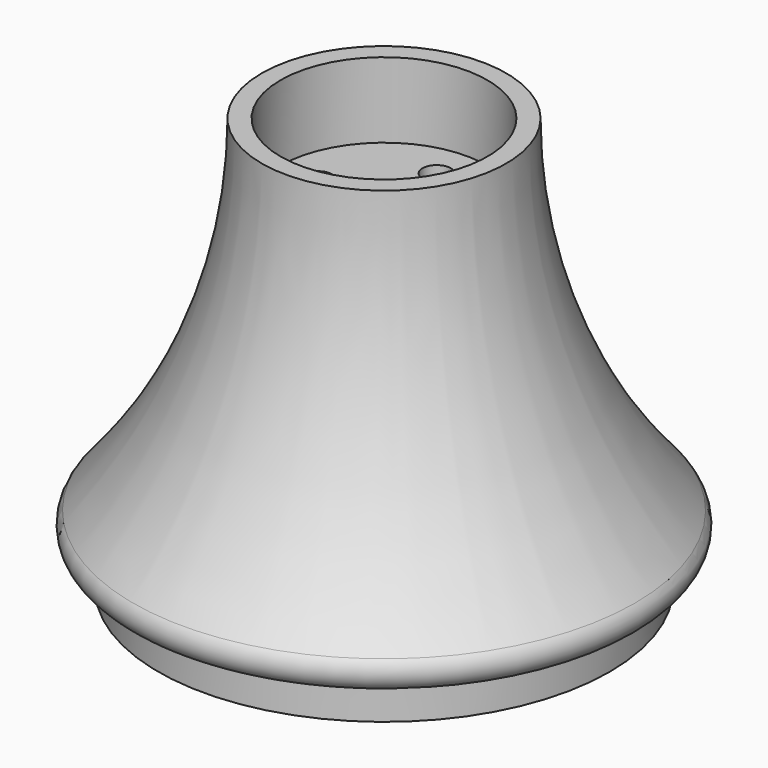
from build123d import *

# Parameters (mm, degrees)
F0_W            = 558.8
F0_H            = 152.4
F2_R            = 152.4
F2_R_2          = 76.2
F3_DEPTH        = 152.4
F3_COPIES_COUNT = 4
F6_DEPTH        = 254


# Not quite as in the source:
# - a pattern or mirror of a feature is missing from the dataset's text; its kind, count and spacing are read off the source's solid


with BuildPart() as f1:
    # F0 (on Front) → F1 (revolve)
    with BuildSketch(Plane.XZ):
        with BuildLine():
            Line((-558.8, -406.4), (-558.8, 0))
            Line((-558.8, 0), (-660.4, 0))
            ThreePointArc((-660.4, 0), (-789.186679788, -846.2615933806), (-1163.8861392232, -1615.9011248632))
            Line((-1163.8861392232, -1615.9011248632), (-1016, -1676.4))
            Line((-1016, -1676.4), (-558.8, -558.8))
            Line((-558.8, -558.8), (-558.8, -406.4))
        make_face()
        with Locations((-279.4, -482.6)):
            Rectangle(F0_W, F0_H)
        with BuildLine():
            Line((-1016, -1676.4), (-1163.8861392232, -1615.9011248632))
            ThreePointArc((-1163.8861392232, -1615.9011248632), (-1256.5295136119, -1742.5177427065), (-1356.0122322887, -1863.8344827586))
            ThreePointArc((-1356.0122322887, -1863.8344827586), (-1371.6828397721, -1972.5871037657), (-1279.255526299, -2032))
            Line((-1279.255526299, -2032), (-1219.2, -2032))
            Line((-1219.2, -2032), (-1219.2, -2235.2))
            Line((-1219.2, -2235.2), (-1016, -2235.2))
            Line((-1016, -2235.2), (-1016, -1676.4))
        make_face()
    revolve(axis=Axis((0, 0, -482.6), (0, 0, -1)))

    # F2 (on face) → F3 (cut)
    with BuildSketch(Plane.XY.offset(-406.4)):
        Circle(F2_R)
        with Locations((0, 355.6)):
            Circle(F2_R_2)
    f3 = extrude(amount=-F3_DEPTH, mode=Mode.SUBTRACT)

    # F3_copies: F3 ×4 about axis
    f3_copies_axis = Axis((0, 0, 0), (0, 0, 1))
    for i in range(1, F3_COPIES_COUNT):
        add(f3.rotate(f3_copies_axis, i * 360 / F3_COPIES_COUNT), mode=Mode.SUBTRACT)

    # F5 (on line) → F6 (cut)
    with BuildSketch(Plane(origin=(-430.7477321435, 0, 176.2149813314), x_dir=(0, -1, 0), z_dir=(-0.9255469562, 0, 0.3786328457))):
        with BuildLine():
            Line((224.0073072261, -1529.8778886352), (0, -1529.8778886352))
            Line((0, -1529.8778886352), (-228.6, -1529.8778886352))
            ThreePointArc((-228.6, -1529.8778886352), (-318.4025612107, -1567.0753274245), (-355.6, -1656.8778886352))
            Line((-355.6, -1656.8778886352), (-355.6, -1743.8760634962))
            ThreePointArc((-355.6, -1743.8760634962), (-317.664288151, -1834.4108776627), (-226.5204318715, -1870.8590363563))
            Line((-226.5204318715, -1870.8590363563), (0, -1867.1493683594))
            Line((0, -1867.1493683594), (227.3898847479, -1863.4254615519))
            ThreePointArc((227.3898847479, -1863.4254615519), (316.5713145497, -1824.7625331708), (352.2932894796, -1734.3629205632))
            Line((352.2932894796, -1734.3629205632), (350.9902800862, -1654.7983205067))
            ThreePointArc((350.9902800862, -1654.7983205067), (313.071595377, -1566.3430744687), (224.0073072261, -1529.8778886352))
        make_face()
    extrude(amount=-F6_DEPTH, mode=Mode.SUBTRACT)


solid = f1.part
